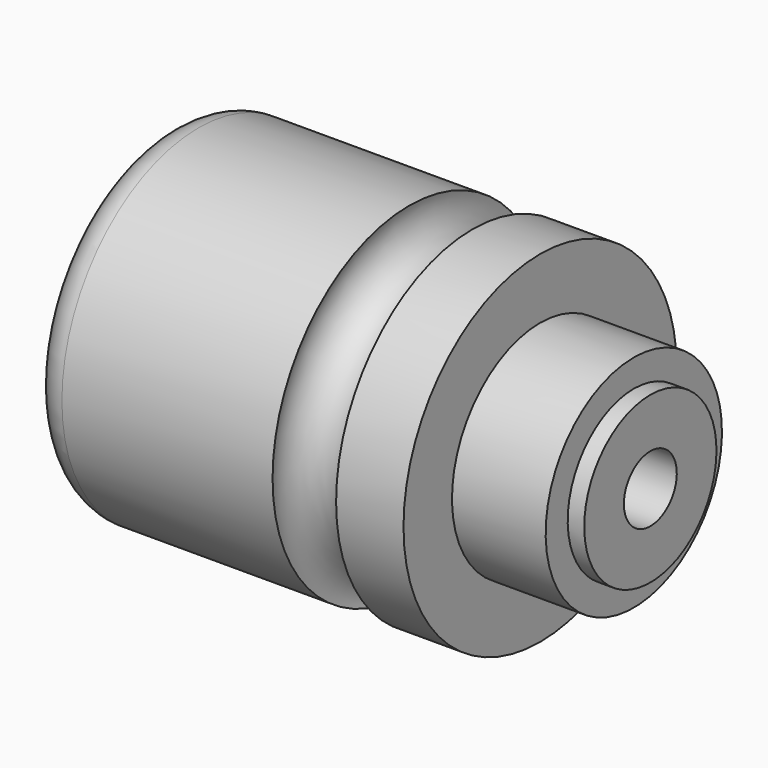
from build123d import *

# Parameters (mm, degrees)
F4_R = 5.99999


# Not quite as in the source:
# - a fillet or chamfer is up to 0.001 mm smaller than in the source, because OpenCascade refuses the exact size


with BuildPart() as f1:
    # F0 (on Front) → F1 (revolve)
    with BuildSketch(Plane.XZ):
        with BuildLine():
            Line((0, 31), (0, 0))
            Line((0, 0), (88, 0))
            Line((88, 0), (88, 15))
            Line((88, 15), (85, 15))
            Line((85, 15), (85, 20))
            Line((85, 20), (68, 20))
            Line((68, 20), (68, 31))
            Line((68, 31), (55.7656139637, 31))
            ThreePointArc((55.7656139637, 31), (50, 23.3393689087), (44.2343860363, 31))
            Line((44.2343860363, 31), (0, 31))
        make_face()
    revolve(axis=Axis((85.9634177689, 0, 0), (1, 0, 0)))

    # F2 (on Front) → F3 (revolve, cut)
    with BuildSketch(Plane.XZ):
        Polygon((0, 25), (0, 0), (88, 0), (88, 6), (30, 6), (30, 12.5), (30, 16), (22, 16), (22, 20.5), (15, 20.5), (15, 12.5), (12, 12.5), (12, 16), (1.5, 16), (1.5, 25), align=None)
    revolve(axis=Axis((-10.4486994627, 0, 0), (-1, 0, 0)), mode=Mode.SUBTRACT)

    # F4 (radius 6 in the source; OpenCascade refuses exactly that, so slightly less here)
    f4_edges = [f1.edges().sort_by_distance(p)[0] for p in [
        (0, 0, -31),
    ]]
    fillet(f4_edges, radius=F4_R)


solid = f1.part
